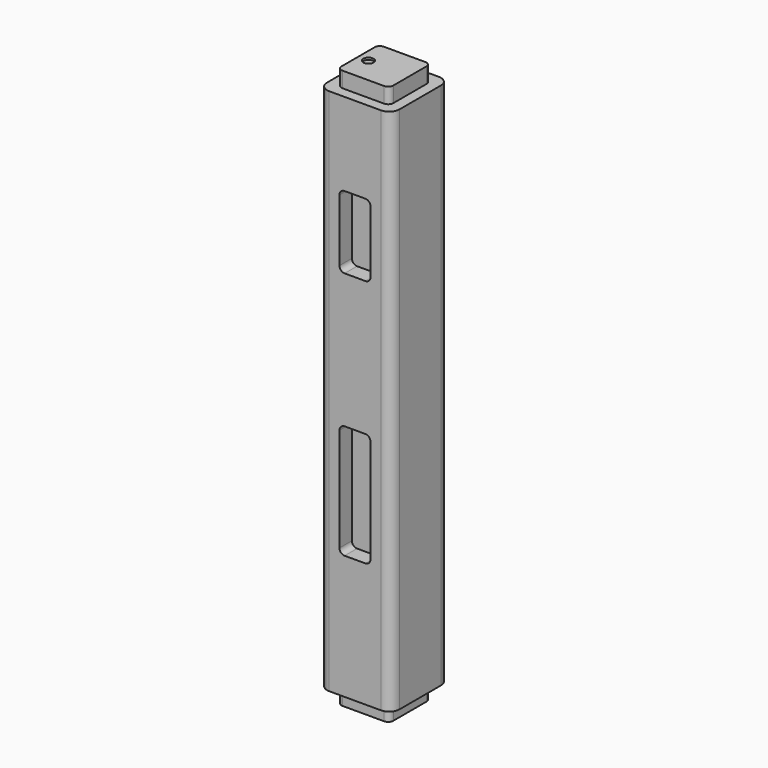
from build123d import *

# Parameters (mm, degrees)
F2_DEPTH  = 647.7
F4_DEPTH  = 19.05
F5_R      = 12.7
F6_R      = 6.35
F7_W      = 38.1
F7_H      = 139.7
F8_DEPTH  = 19.05
F9_R      = 6.35
F11_DEPTH = 19.05
F13_DEPTH = 19.05
F14_R     = 6.35
F15_DEPTH = 2.54


with BuildPart() as f2:
    # F1 (on Top) → F2 (new body)
    with BuildSketch(Plane.XY):
        Polygon((-44.45, 19.05), (-44.45, 0), (-44.45, -19.05), (-44.45, -44.45), (-19.05, -44.45), (0, -44.45), (19.05, -44.45), (44.45, -44.45), (44.45, -19.05), (44.45, 0), (44.45, 19.05), (44.45, 44.45), (19.05, 44.45), (0, 44.45), (-19.05, 44.45), (-44.45, 44.45), align=None)
    extrude(amount=-F2_DEPTH)

    # F3 (on face) → F4 (cut)
    with BuildSketch(Plane.XZ.offset(44.45)):
        Polygon((19.05, -101.6), (-19.05, -101.6), (-19.05, -190.5), (0, -190.5), (19.05, -190.5), align=None)
    extrude(amount=-F4_DEPTH, mode=Mode.SUBTRACT)

    # F5
    f5_edges = [f2.edges().sort_by_distance(p)[0] for p in [
        (-44.45, -44.45, -323.85),
        (44.45, -44.45, -323.85),
        (44.45, 44.45, -323.85),
        (-44.45, 44.45, -323.85),
    ]]
    fillet(f5_edges, radius=F5_R)

    # F6
    f6_edges = [f2.edges().sort_by_distance(p)[0] for p in [
        (-19.05, -34.925, -190.5),
        (19.05, -34.925, -190.5),
        (-19.05, -34.925, -101.6),
        (19.05, -34.925, -101.6),
    ]]
    fillet(f6_edges, radius=F6_R)

    # F7 (on face) → F8 (cut)
    with BuildSketch(Plane.XZ.offset(44.45)):
        with Locations((0, -425.45)):
            Rectangle(F7_W, F7_H)
    extrude(amount=-F8_DEPTH, mode=Mode.SUBTRACT)

    # F9
    f9_edges = [f2.edges().sort_by_distance(p)[0] for p in [
        (-19.05, -34.925, -355.6),
        (19.05, -34.925, -355.6),
        (19.05, -34.925, -495.3),
        (-19.05, -34.925, -495.3),
    ]]
    fillet(f9_edges, radius=F9_R)

    # F10 (on face) → F11 (join)
    with BuildSketch(Plane.XY):
        with BuildLine():
            Line((-25.4, -31.75), (25.4, -31.75))
            ThreePointArc((25.4, -31.75), (29.8901280605, -29.8901280605), (31.75, -25.4))
            Line((31.75, -25.4), (31.75, 25.4))
            ThreePointArc((31.75, 25.4), (29.8901280605, 29.8901280605), (25.4, 31.75))
            Line((25.4, 31.75), (-25.4, 31.75))
            ThreePointArc((-25.4, 31.75), (-29.8901280605, 29.8901280605), (-31.75, 25.4))
            Line((-31.75, 25.4), (-31.75, -25.4))
            ThreePointArc((-31.75, -25.4), (-29.8901280605, -29.8901280605), (-25.4, -31.75))
        make_face()
    extrude(amount=F11_DEPTH)

    # F12 (on face) → F13 (join)
    with BuildSketch(Plane(origin=(0, 0, -647.7), x_dir=(1, 0, 0), z_dir=(0, 0, -1))):
        with BuildLine():
            Line((-25.4, -31.75), (25.4, -31.75))
            ThreePointArc((25.4, -31.75), (29.8901280605, -29.8901280605), (31.75, -25.4))
            Line((31.75, -25.4), (31.75, 25.4))
            ThreePointArc((31.75, 25.4), (29.8901280605, 29.8901280605), (25.4, 31.75))
            Line((25.4, 31.75), (-25.4, 31.75))
            ThreePointArc((-25.4, 31.75), (-29.8901280605, 29.8901280605), (-31.75, 25.4))
            Line((-31.75, 25.4), (-31.75, -25.4))
            ThreePointArc((-31.75, -25.4), (-29.8901280605, -29.8901280605), (-25.4, -31.75))
        make_face()
    extrude(amount=F13_DEPTH)

    # F14 (on face) → F15 (cut)
    with BuildSketch(Plane.XY.offset(19.05)):
        with Locations((-19.05, 0)):
            Circle(F14_R)
    extrude(amount=-F15_DEPTH, mode=Mode.SUBTRACT)


solid = f2.part
